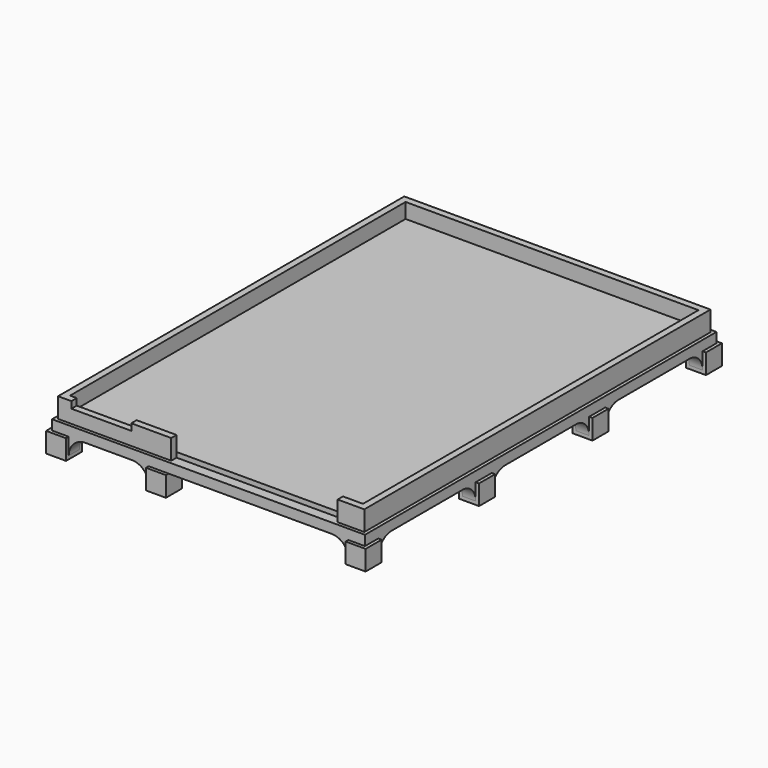
from build123d import *

# Parameters (mm, degrees)
F0_W      = 4700
F0_H      = 6600
F0_W_2    = 4300
F0_H_2    = 6200
F1_DEPTH  = 150
F2_W      = 4600
F2_H      = 6500
F2_W_2    = 4400
F2_H_2    = 6300
F3_DEPTH  = 300
F4_W      = 300
F4_H      = 300
F5_DEPTH  = 300
F6_W      = 2500
F6_H      = 500
F7_DEPTH  = 500
F9_W      = 4400
F9_H      = 6300
F10_DEPTH = 125
F11_R     = 250
F12_W     = 900
F12_H     = 100
F13_DEPTH = 100


with BuildPart() as f1:
    # F0 (on Top) → F1 (new body)
    with BuildSketch(Plane.XY):
        Rectangle(F0_W, F0_H)
        Rectangle(F0_W_2, F0_H_2, mode=Mode.SUBTRACT)
    extrude(amount=F1_DEPTH)

    # F2 (on face) → F3 (join)
    with BuildSketch(Plane.XY.offset(150)):
        Rectangle(F2_W, F2_H)
        Rectangle(F2_W_2, F2_H_2, mode=Mode.SUBTRACT)
    extrude(amount=F3_DEPTH)

    # F4 (on Top) → F5 (join)
    with BuildSketch(Plane.XY):
        with Locations((-2250, -3200)):
            Rectangle(F4_W, F4_H)
        with Locations((-2250, -1070)):
            Rectangle(F4_W, F4_H)
        with Locations((2250, -3200)):
            Rectangle(F4_W, F4_H)
        with Locations((2250, -1070)):
            Rectangle(F4_W, F4_H)
        with Locations((-2250, 1060)):
            Rectangle(F4_W, F4_H)
        with Locations((-2250, 3190)):
            Rectangle(F4_W, F4_H)
        with Locations((2250, 1060)):
            Rectangle(F4_W, F4_H)
        with Locations((2250, 3190)):
            Rectangle(F4_W, F4_H)
        with Locations((-750, -3200)):
            Rectangle(F4_W, F4_H)
    extrude(amount=-F5_DEPTH)

    # F6 (on face) + F1_face2 (on face) → F7 (cut)
    with BuildSketch(Plane.XZ.offset(3300)):
        with Locations((650, 400)):
            Rectangle(F6_W, F6_H)
    with BuildSketch(Plane(origin=(0, -3100, 75), x_dir=(-1, 0, 0), z_dir=(0, 1, 0))):
        Polygon((-2150, 75), (-2150, -75), (-2100, -75), (600, -75), (900, -75), (2100, -75), (2150, -75), (2150, 75), align=None)
    extrude(amount=-F7_DEPTH, dir=(0, -1, 0), mode=Mode.SUBTRACT)

    # F11
    f11_edges = [f1.edges().sort_by_distance(p)[0] for p in [
        (-2100, 3200, 0),
        (-2250, 3040, 0),
        (-2250, 1210, 0),
        (-2250, 910, 0),
        (-2250, -1220, 0),
        (-2250, -920, 0),
        (-2250, -3050, 0),
        (-900, -3200, 0),
        (-2100, -3200, 0),
        (2100, -3200, 0),
        (2250, -1220, 0),
        (2250, 910, 0),
        (2250, 3040, 0),
        (2100, 3200, 0),
        (2250, -3050, 0),
        (2250, -920, 0),
        (2250, 1210, 0),
    ]]
    fillet(f11_edges, radius=F11_R)

    # F12 (on face) → F13 (cut, through all)
    with BuildSketch(Plane.XZ.offset(3250)):
        with Locations((-1650, 400)):
            Rectangle(F12_W, F12_H)
    extrude(amount=-F13_DEPTH, mode=Mode.SUBTRACT)


with BuildPart() as f10:
    # F9 (on offset) → F10 (new body)
    with BuildSketch(Plane.XY.offset(100)):
        Rectangle(F9_W, F9_H)
    extrude(amount=F10_DEPTH)


solid = Compound([f1.part, f10.part])
